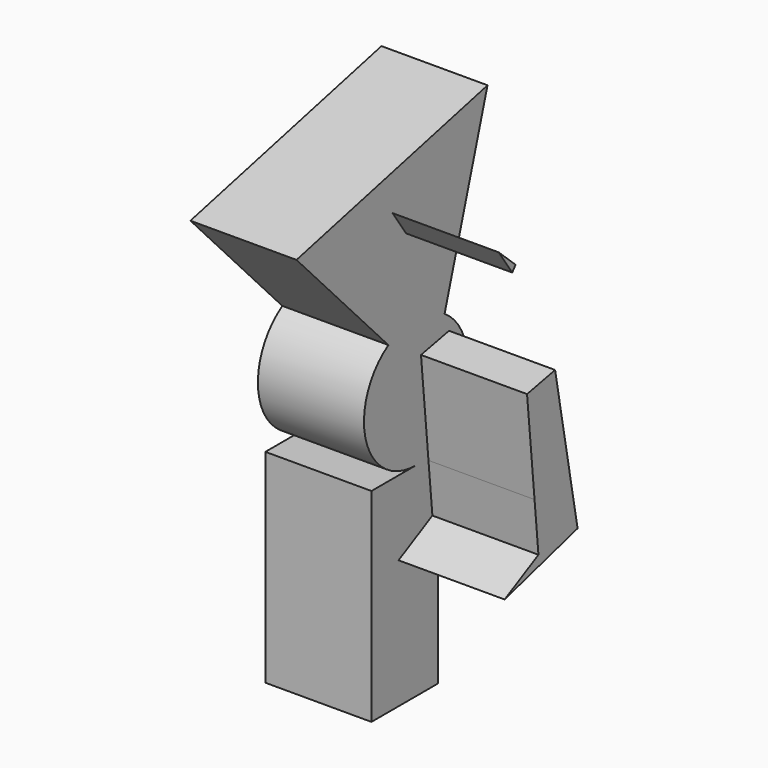
from build123d import *

# Parameters (mm, degrees)
F1_DEPTH = 25.4
F3_DEPTH = 25.4


with BuildPart() as f1:
    # F0 (on Right) → F1 (new body)
    with BuildSketch(Plane.YZ):
        Polygon((-13.2883740589, -47.1408768902), (-13.2883740589, -64.2038285732), (6.5742493607, -64.2038285732), (6.5742493607, -19.7971570041), (0, -15.5264167115), (-13.2883740589, -15.5264167115), align=None)
        Polygon((0, -15.5264167115), (6.5742493607, -19.7971570041), (6.5742493607, -15.5264167115), align=None)
        with BuildLine():
            Line((0, -15.5264167115), (6.5742493607, -15.5264167115))
            Line((6.5742493607, -15.5264167115), (8.9490753187, -12.6879339074))
            ThreePointArc((8.9490753187, -12.6879339074), (4.6942234099, -14.7997933255), (0, -15.5264167115))
        make_face()
        with BuildLine():
            ThreePointArc((-8.216208845, 13.1743511459), (-14.9268228651, -4.2731224008), (0, -15.5264167115))
            ThreePointArc((0, -15.5264167115), (4.6942234099, -14.7997933255), (8.9490753187, -12.6879339074))
            Line((8.9490753187, -12.6879339074), (14.0681090783, -6.5694689939))
            ThreePointArc((14.0681090783, -6.5694689939), (15.1574559177, -3.3646910711), (15.5264167115, 0))
            ThreePointArc((15.5264167115, 0), (13.6875468883, 7.3294390017), (8.6065101962, 12.9227550523))
            Line((8.6065101962, 12.9227550523), (4.6159664635, -0.419639051))
            Line((4.6159664635, -0.419639051), (-8.216208845, 13.1743511459))
        make_face()
        with BuildLine():
            Line((14.0681090783, -6.5694689939), (8.9490753187, -12.6879339074))
            ThreePointArc((8.9490753187, -12.6879339074), (11.908257539, -9.9630827701), (14.0681090783, -6.5694689939))
        make_face()
        with BuildLine():
            Line((-35.7222311496, 42.3133387746), (-8.216208845, 13.1743511459))
            ThreePointArc((-8.216208845, 13.1743511459), (0.2321829769, 15.5246805753), (8.6065101962, 12.9227550523))
            Line((8.6065101962, 12.9227550523), (21.4547120332, 55.8807537376))
            Line((21.4547120332, 55.8807537376), (-35.7222311496, 42.3133387746))
        make_face()
        with BuildLine():
            ThreePointArc((8.6065101962, 12.9227550523), (0.2321829769, 15.5246805753), (-8.216208845, 13.1743511459))
            Line((-8.216208845, 13.1743511459), (4.6159664635, -0.419639051))
            Line((4.6159664635, -0.419639051), (8.6065101962, 12.9227550523))
        make_face()
    extrude(amount=F1_DEPTH)

    # F2 (on face) → F3 (join)
    with BuildSketch(Plane.YZ.offset(25.4)):
        Polygon((-2.8975114851, 34.5519260837), (-1.9047569793, 35.8120341569), (-6.9570055408, 40.475821833), align=None)
        Polygon((9.9313091487, 8.8122906163), (1.5386517625, 7.1337586269), (3.7782862439, -16.0091173098), (14.0347183236, -13.2288791008), align=None)
        Polygon((14.0347183236, -13.2288791008), (3.7782862439, -16.0091173098), (4.9502783877, -28.1196956248), (15.7521614301, -22.4540022549), align=None)
        Polygon((15.7521614301, -22.4540022549), (4.9502783877, -28.1196956248), (5.1841876849, -30.5367569319), (16.6601009867, -27.330934827), align=None)
        Polygon((5.1841876849, -30.5367569319), (4.9502783877, -28.1196956248), (-5.1754731685, -33.4307514131), align=None)
    extrude(amount=F3_DEPTH)


solid = f1.part
